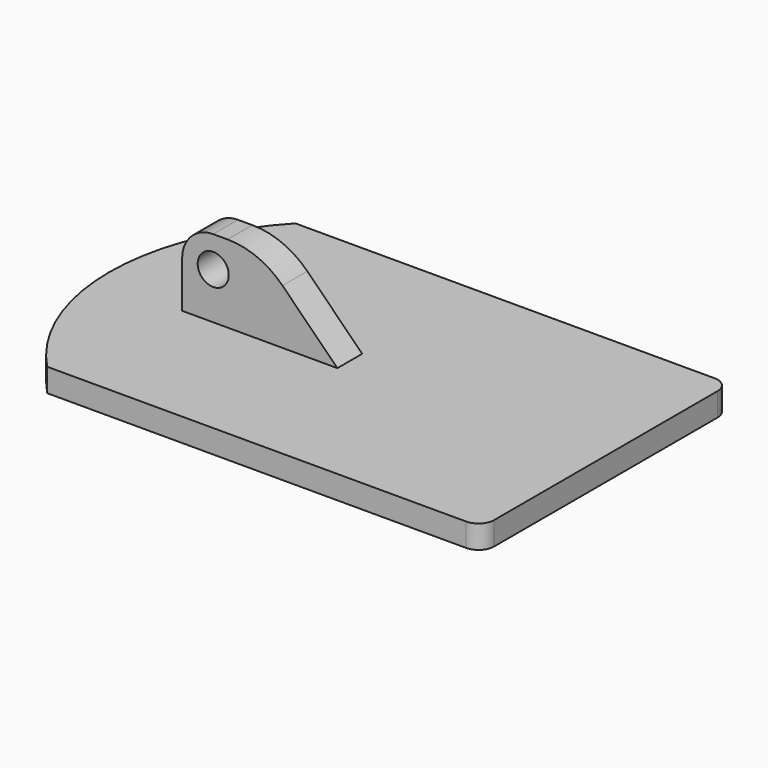
from build123d import *

# Parameters (mm, degrees)
F0_W      = 28
F0_H      = 20
F1_DEPTH  = 1.5
F2_R      = 1
F3_W      = 10
F3_H      = 1
F4_DEPTH  = 5
F5_R      = 2
F6_SIZE   = 4.99999
F7_R      = 5
F9_R      = 1
F10_DEPTH = 25
F12_DEPTH = 1.5


# Not quite as in the source:
# - a fillet or chamfer is up to 0.001 mm smaller than in the source, because OpenCascade refuses the exact size


with BuildPart() as f1:
    # F0 (on Top) → F1 (new body)
    with BuildSketch(Plane.XY):
        Rectangle(F0_W, F0_H)
    extrude(amount=F1_DEPTH)

    # F2
    f2_edges = [f1.edges().sort_by_distance(p)[0] for p in [
        (14, -10, 0.75),
        (14, 10, 0.75),
    ]]
    fillet(f2_edges, radius=F2_R)



with BuildPart() as f4:
    # F3 (on face) → F4 (new body)
    with BuildSketch(Plane.XY.offset(1.5)):
        with Locations((-7.5, 0.5)):
            Rectangle(F3_W, F3_H)
    extrude(amount=F4_DEPTH)

    # F5
    f5_edges = [f4.edges().sort_by_distance(p)[0] for p in [
        (-12.5, 0.5, 6.5),
    ]]
    fillet(f5_edges, radius=F5_R)

    # F6 (size 5 in the source; OpenCascade refuses exactly that, so slightly less here)
    f6_edges = [f4.edges().sort_by_distance(p)[0] for p in [
        (-2.5, 0.5, 6.5),
    ]]
    chamfer(f6_edges, length=F6_SIZE)

    # F7
    f7_edges = [f4.edges().sort_by_distance(p)[0] for p in [
        (-7.49999, 0.5, 6.5),
    ]]
    fillet(f7_edges, radius=F7_R)


with BuildPart() as f1_1:
    add(f1.part)

    add(f4.part)  # F8 merges F4
    # F8: F4 across plane
    add(f4.part.mirror(Plane.XZ))

    # F9 (on face) → F10 (cut)
    with BuildSketch(Plane.XZ.offset(1)):
        with Locations((-10.5, 4.5)):
            Circle(F9_R)
    extrude(amount=-F10_DEPTH, mode=Mode.SUBTRACT)

    # F11 (on face) → F12 (join)
    with BuildSketch(Plane(origin=(0, 0, 0), x_dir=(1, 0, 0), z_dir=(0, 0, -1))):
        with BuildLine():
            Line((-14, -10), (-14, 10))
            ThreePointArc((-14, 10), (-18, 0), (-14, -10))
        make_face()
    extrude(amount=-F12_DEPTH)


solid = f1_1.part
